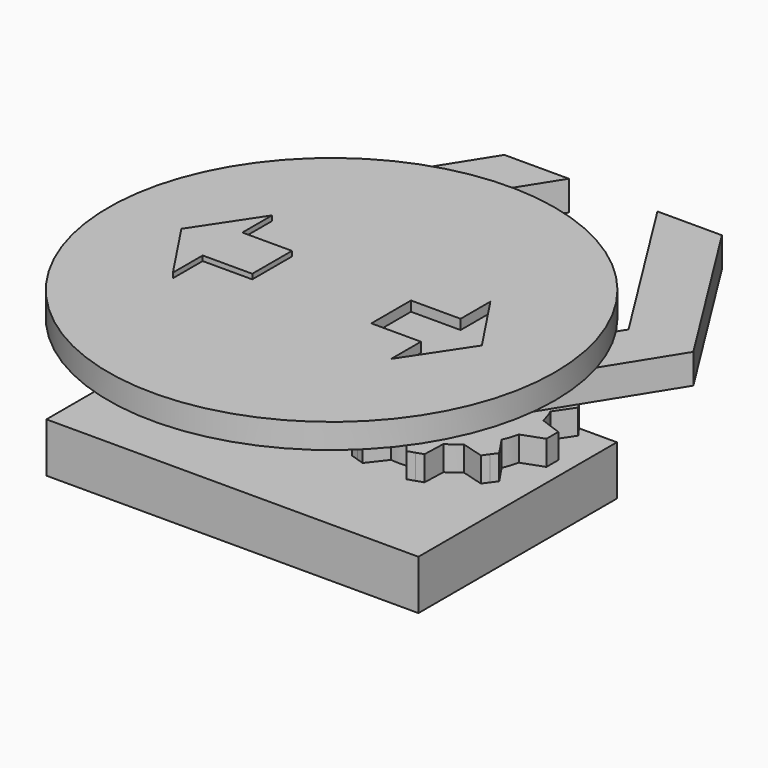
from build123d import *

# Parameters (mm, degrees)
F0_W      = 75
F0_H      = 50
F1_DEPTH  = 10
F2_R      = 10
F2_R_2    = 3.5
F3_DEPTH  = 2
F4_DEPTH  = 20
F5_DEPTH  = 20
F7_DEPTH  = 5
F9_DEPTH  = 5
F10_R     = 3.5
F11_DEPTH = 6
F13_R     = 45
F14_DEPTH = 5
F15_R     = 5
F15_R_2   = 3.5
F16_DEPTH = 7
F18_DEPTH = 2
F19_DEPTH = 3


with BuildPart() as f1:
    # F0 (on Top) → F1 (new body)
    with BuildSketch(Plane.XY):
        Rectangle(F0_W, F0_H)
    extrude(amount=F1_DEPTH)

    # F2 (on face) → F3 (join)
    with BuildSketch(Plane.XY.offset(10)):
        with Locations((-17.5, 10)):
            Circle(F2_R)
        with Locations((-17.5, 10)):
            Circle(F2_R_2, mode=Mode.SUBTRACT)
        with Locations((17.5, 10)):
            Circle(F2_R)
        with Locations((17.5, 10)):
            Circle(F2_R_2, mode=Mode.SUBTRACT)
    extrude(amount=F3_DEPTH)


with BuildPart() as f4:
    # F4 (new): a face of the model
    f4_faces = [f1.part.faces().sort_by_distance(p)[0] for p in [
        (-17.5, 10, 10),
    ]]
    extrude(f4_faces, amount=F4_DEPTH)

    # F6 (on face) → F7 (join)
    with BuildSketch(Plane.XY.offset(12)):
        with BuildLine():
            ThreePointArc((-2.587280565, 8.3842032761), (-2.521836035, 9.190923837), (-2.5, 10))
            ThreePointArc((-2.5, 10), (-2.521836035, 10.809076163), (-2.587280565, 11.6157967239))
            ThreePointArc((-2.587280565, 11.6157967239), (-3.2341522556, 14.6352549156), (-4.4856150597, 17.4582695463))
            ThreePointArc((-4.4856150597, 17.4582695463), (-5.3647450844, 18.8167787844), (-6.3850980298, 20.0726835646))
            ThreePointArc((-6.3850980298, 20.0726835646), (-8.6832212156, 22.1352549156), (-11.3550022589, 23.6835303472))
            ThreePointArc((-11.3550022589, 23.6835303472), (-12.8647450844, 24.2658477444), (-14.4284302655, 24.6821476415))
            ThreePointArc((-14.4284302655, 24.6821476415), (-17.5, 25), (-20.5715697345, 24.6821476415))
            ThreePointArc((-20.5715697345, 24.6821476415), (-22.1352549156, 24.2658477444), (-23.6449977411, 23.6835303472))
            ThreePointArc((-23.6449977411, 23.6835303472), (-26.3167787844, 22.1352549156), (-28.6149019702, 20.0726835646))
            ThreePointArc((-28.6149019702, 20.0726835646), (-29.6352549156, 18.8167787844), (-30.5143849403, 17.4582695463))
            ThreePointArc((-30.5143849403, 17.4582695463), (-31.7658477444, 14.6352549156), (-32.412719435, 11.6157967239))
            ThreePointArc((-32.412719435, 11.6157967239), (-32.5, 10), (-32.412719435, 8.3842032761))
            ThreePointArc((-32.412719435, 8.3842032761), (-31.7658477444, 5.3647450844), (-30.5143849403, 2.5417304537))
            ThreePointArc((-30.5143849403, 2.5417304537), (-29.6352549156, 1.1832212156), (-28.6149019702, -0.0726835646))
            ThreePointArc((-28.6149019702, -0.0726835646), (-26.3167787844, -2.1352549156), (-23.6449977411, -3.6835303472))
            ThreePointArc((-23.6449977411, -3.6835303472), (-22.1352549156, -4.2658477444), (-20.5715697345, -4.6821476415))
            ThreePointArc((-20.5715697345, -4.6821476415), (-17.5, -5), (-14.4284302655, -4.6821476415))
            ThreePointArc((-14.4284302655, -4.6821476415), (-12.8647450844, -4.2658477444), (-11.3550022589, -3.6835303472))
            ThreePointArc((-11.3550022589, -3.6835303472), (-8.6832212156, -2.1352549156), (-6.3850980298, -0.0726835646))
            ThreePointArc((-6.3850980298, -0.0726835646), (-5.3647450844, 1.1832212156), (-4.4856150597, 2.5417304537))
            ThreePointArc((-4.4856150597, 2.5417304537), (-3.2341522556, 5.3647450844), (-2.587280565, 8.3842032761))
        make_face()
        with BuildLine():
            ThreePointArc((-4.4856150597, 17.4582695463), (-3.2341522556, 14.6352549156), (-2.587280565, 11.6157967239))
            Line((-2.587280565, 11.6157967239), (1.0335993012, 14.4447381187))
            Line((1.0335993012, 14.4447381187), (0.5700738096, 15.8713228931))
            Line((0.5700738096, 15.8713228931), (0.106548318, 17.2979076676))
            Line((0.106548318, 17.2979076676), (-4.4856150597, 17.4582695463))
        make_face()
        with BuildLine():
            Line((1.0335993012, 5.5552618813), (-2.587280565, 8.3842032761))
            ThreePointArc((-2.587280565, 8.3842032761), (-3.2341522556, 5.3647450844), (-4.4856150597, 2.5417304537))
            Line((-4.4856150597, 2.5417304537), (0.106548318, 2.7020923324))
            Line((0.106548318, 2.7020923324), (0.5700738096, 4.1286771069))
            Line((0.5700738096, 4.1286771069), (1.0335993012, 5.5552618813))
        make_face()
        with BuildLine():
            ThreePointArc((-11.3550022589, 23.6835303472), (-8.6832212156, 22.1352549156), (-6.3850980298, 20.0726835646))
            Line((-6.3850980298, 20.0726835646), (-5.1185547149, 24.4896450147))
            Line((-5.1185547149, 24.4896450147), (-6.3320802064, 25.3713228931))
            Line((-6.3320802064, 25.3713228931), (-7.545605698, 26.2530007716))
            Line((-7.545605698, 26.2530007716), (-11.3550022589, 23.6835303472))
        make_face()
        with BuildLine():
            Line((-5.1185547149, -4.4896450147), (-6.3850980298, -0.0726835646))
            ThreePointArc((-6.3850980298, -0.0726835646), (-8.6832212156, -2.1352549156), (-11.3550022589, -3.6835303472))
            Line((-11.3550022589, -3.6835303472), (-7.545605698, -6.2530007716))
            Line((-7.545605698, -6.2530007716), (-6.3320802064, -5.3713228931))
            Line((-6.3320802064, -5.3713228931), (-5.1185547149, -4.4896450147))
        make_face()
        with BuildLine():
            ThreePointArc((-20.5715697345, 24.6821476415), (-17.5, 25), (-14.4284302655, 24.6821476415))
            Line((-14.4284302655, 24.6821476415), (-16, 29))
            Line((-16, 29), (-17.5, 29))
            Line((-17.5, 29), (-19, 29))
            Line((-19, 29), (-20.5715697345, 24.6821476415))
        make_face()
        with BuildLine():
            Line((-16, -9), (-14.4284302655, -4.6821476415))
            ThreePointArc((-14.4284302655, -4.6821476415), (-17.5, -5), (-20.5715697345, -4.6821476415))
            Line((-20.5715697345, -4.6821476415), (-19, -9))
            Line((-19, -9), (-17.5, -9))
            Line((-17.5, -9), (-16, -9))
        make_face()
        with BuildLine():
            ThreePointArc((-28.6149019702, 20.0726835646), (-26.3167787844, 22.1352549156), (-23.6449977411, 23.6835303472))
            Line((-23.6449977411, 23.6835303472), (-27.454394302, 26.2530007716))
            Line((-27.454394302, 26.2530007716), (-28.6679197936, 25.3713228931))
            Line((-28.6679197936, 25.3713228931), (-29.8814452851, 24.4896450147))
            Line((-29.8814452851, 24.4896450147), (-28.6149019702, 20.0726835646))
        make_face()
        with BuildLine():
            Line((-27.454394302, -6.2530007716), (-23.6449977411, -3.6835303472))
            ThreePointArc((-23.6449977411, -3.6835303472), (-26.3167787844, -2.1352549156), (-28.6149019702, -0.0726835646))
            Line((-28.6149019702, -0.0726835646), (-29.8814452851, -4.4896450147))
            Line((-29.8814452851, -4.4896450147), (-28.6679197936, -5.3713228931))
            Line((-28.6679197936, -5.3713228931), (-27.454394302, -6.2530007716))
        make_face()
        with BuildLine():
            ThreePointArc((-32.412719435, 11.6157967239), (-31.7658477444, 14.6352549156), (-30.5143849403, 17.4582695463))
            Line((-30.5143849403, 17.4582695463), (-35.106548318, 17.2979076676))
            Line((-35.106548318, 17.2979076676), (-35.5700738096, 15.8713228931))
            Line((-35.5700738096, 15.8713228931), (-36.0335993012, 14.4447381187))
            Line((-36.0335993012, 14.4447381187), (-32.412719435, 11.6157967239))
        make_face()
        with BuildLine():
            Line((-35.106548318, 2.7020923324), (-30.5143849403, 2.5417304537))
            ThreePointArc((-30.5143849403, 2.5417304537), (-31.7658477444, 5.3647450844), (-32.412719435, 8.3842032761))
            Line((-32.412719435, 8.3842032761), (-36.0335993012, 5.5552618813))
            Line((-36.0335993012, 5.5552618813), (-35.5700738096, 4.1286771069))
            Line((-35.5700738096, 4.1286771069), (-35.106548318, 2.7020923324))
        make_face()
    extrude(amount=F7_DEPTH)


with BuildPart() as f5:
    # F5 (new): a face of the model
    f5_faces = [f1.part.faces().sort_by_distance(p)[0] for p in [
        (17.5, 10, 10),
    ]]
    extrude(f5_faces, amount=F5_DEPTH)

    # F8 (on face) → F9 (join)
    with BuildSketch(Plane.XY.offset(12)):
        with BuildLine():
            ThreePointArc((32.1821476415, 6.9284302655), (32.4203253085, 8.4560140257), (32.5, 10))
            ThreePointArc((32.5, 10), (32.4203253085, 11.5439859743), (32.1821476415, 13.0715697345))
            ThreePointArc((32.1821476415, 13.0715697345), (31.7658477444, 14.6352549156), (31.1835303472, 16.1449977411))
            ThreePointArc((31.1835303472, 16.1449977411), (29.6352549156, 18.8167787844), (27.5726835646, 21.1149019702))
            ThreePointArc((27.5726835646, 21.1149019702), (26.3167787844, 22.1352549156), (24.9582695463, 23.0143849403))
            ThreePointArc((24.9582695463, 23.0143849403), (22.1352549156, 24.2658477444), (19.1157967239, 24.912719435))
            ThreePointArc((19.1157967239, 24.912719435), (17.5, 25), (15.8842032761, 24.912719435))
            ThreePointArc((15.8842032761, 24.912719435), (12.8647450844, 24.2658477444), (10.0417304537, 23.0143849403))
            ThreePointArc((10.0417304537, 23.0143849403), (8.6832212156, 22.1352549156), (7.4273164354, 21.1149019702))
            ThreePointArc((7.4273164354, 21.1149019702), (5.3647450844, 18.8167787844), (3.8164696528, 16.1449977411))
            ThreePointArc((3.8164696528, 16.1449977411), (3.2341522556, 14.6352549156), (2.8178523585, 13.0715697345))
            ThreePointArc((2.8178523585, 13.0715697345), (2.5, 10), (2.8178523585, 6.9284302655))
            ThreePointArc((2.8178523585, 6.9284302655), (3.2341522556, 5.3647450844), (3.8164696528, 3.8550022589))
            ThreePointArc((3.8164696528, 3.8550022589), (5.3647450844, 1.1832212156), (7.4273164354, -1.1149019702))
            ThreePointArc((7.4273164354, -1.1149019702), (8.6832212156, -2.1352549156), (10.0417304537, -3.0143849403))
            ThreePointArc((10.0417304537, -3.0143849403), (12.8647450844, -4.2658477444), (15.8842032761, -4.912719435))
            ThreePointArc((15.8842032761, -4.912719435), (17.5, -5), (19.1157967239, -4.912719435))
            ThreePointArc((19.1157967239, -4.912719435), (22.1352549156, -4.2658477444), (24.9582695463, -3.0143849403))
            ThreePointArc((24.9582695463, -3.0143849403), (26.3167787844, -2.1352549156), (27.5726835646, -1.1149019702))
            ThreePointArc((27.5726835646, -1.1149019702), (29.6352549156, 1.1832212156), (31.1835303472, 3.8550022589))
            ThreePointArc((31.1835303472, 3.8550022589), (31.7658477444, 5.3647450844), (32.1821476415, 6.9284302655))
        make_face()
        with BuildLine():
            ThreePointArc((32.1821476415, 13.0715697345), (32.4203253085, 11.5439859743), (32.5, 10))
            ThreePointArc((32.5, 10), (32.4203253085, 8.4560140257), (32.1821476415, 6.9284302655))
            Line((32.1821476415, 6.9284302655), (36.5, 8.5))
            Line((36.5, 8.5), (36.5, 10))
            Line((36.5, 10), (36.5, 11.5))
            Line((36.5, 11.5), (32.1821476415, 13.0715697345))
        make_face()
        with BuildLine():
            ThreePointArc((27.5726835646, 21.1149019702), (29.6352549156, 18.8167787844), (31.1835303472, 16.1449977411))
            Line((31.1835303472, 16.1449977411), (33.7530007716, 19.954394302))
            Line((33.7530007716, 19.954394302), (32.8713228931, 21.1679197936))
            Line((32.8713228931, 21.1679197936), (31.9896450147, 22.3814452851))
            Line((31.9896450147, 22.3814452851), (27.5726835646, 21.1149019702))
        make_face()
        with BuildLine():
            Line((33.7530007716, 0.045605698), (31.1835303472, 3.8550022589))
            ThreePointArc((31.1835303472, 3.8550022589), (29.6352549156, 1.1832212156), (27.5726835646, -1.1149019702))
            Line((27.5726835646, -1.1149019702), (31.9896450147, -2.3814452851))
            Line((31.9896450147, -2.3814452851), (32.8713228931, -1.1679197936))
            Line((32.8713228931, -1.1679197936), (33.7530007716, 0.045605698))
        make_face()
        with BuildLine():
            ThreePointArc((19.1157967239, 24.912719435), (22.1352549156, 24.2658477444), (24.9582695463, 23.0143849403))
            Line((24.9582695463, 23.0143849403), (24.7979076676, 27.606548318))
            Line((24.7979076676, 27.606548318), (23.3713228931, 28.0700738096))
            Line((23.3713228931, 28.0700738096), (21.9447381187, 28.5335993012))
            Line((21.9447381187, 28.5335993012), (19.1157967239, 24.912719435))
        make_face()
        with BuildLine():
            Line((24.7979076676, -7.606548318), (24.9582695463, -3.0143849403))
            ThreePointArc((24.9582695463, -3.0143849403), (22.1352549156, -4.2658477444), (19.1157967239, -4.912719435))
            Line((19.1157967239, -4.912719435), (21.9447381187, -8.5335993012))
            Line((21.9447381187, -8.5335993012), (23.3713228931, -8.0700738096))
            Line((23.3713228931, -8.0700738096), (24.7979076676, -7.606548318))
        make_face()
        with BuildLine():
            ThreePointArc((10.0417304537, 23.0143849403), (12.8647450844, 24.2658477444), (15.8842032761, 24.912719435))
            Line((15.8842032761, 24.912719435), (13.0552618813, 28.5335993012))
            Line((13.0552618813, 28.5335993012), (11.6286771069, 28.0700738096))
            Line((11.6286771069, 28.0700738096), (10.2020923324, 27.606548318))
            Line((10.2020923324, 27.606548318), (10.0417304537, 23.0143849403))
        make_face()
        with BuildLine():
            Line((13.0552618813, -8.5335993012), (15.8842032761, -4.912719435))
            ThreePointArc((15.8842032761, -4.912719435), (12.8647450844, -4.2658477444), (10.0417304537, -3.0143849403))
            Line((10.0417304537, -3.0143849403), (10.2020923324, -7.606548318))
            Line((10.2020923324, -7.606548318), (11.6286771069, -8.0700738096))
            Line((11.6286771069, -8.0700738096), (13.0552618813, -8.5335993012))
        make_face()
        with BuildLine():
            ThreePointArc((3.8164696528, 16.1449977411), (5.3647450844, 18.8167787844), (7.4273164354, 21.1149019702))
            Line((7.4273164354, 21.1149019702), (3.0103549853, 22.3814452851))
            Line((3.0103549853, 22.3814452851), (2.1286771069, 21.1679197936))
            Line((2.1286771069, 21.1679197936), (1.2469992284, 19.954394302))
            Line((1.2469992284, 19.954394302), (3.8164696528, 16.1449977411))
        make_face()
        with BuildLine():
            Line((3.0103549853, -2.3814452851), (7.4273164354, -1.1149019702))
            ThreePointArc((7.4273164354, -1.1149019702), (5.3647450844, 1.1832212156), (3.8164696528, 3.8550022589))
            Line((3.8164696528, 3.8550022589), (1.2469992284, 0.045605698))
            Line((1.2469992284, 0.045605698), (2.1286771069, -1.1679197936))
            Line((2.1286771069, -1.1679197936), (3.0103549853, -2.3814452851))
        make_face()
        with BuildLine():
            ThreePointArc((2.8178523585, 6.9284302655), (2.5, 10), (2.8178523585, 13.0715697345))
            Line((2.8178523585, 13.0715697345), (-1.5, 11.5))
            Line((-1.5, 11.5), (-1.5, 10))
            Line((-1.5, 10), (-1.5, 8.5))
            Line((-1.5, 8.5), (2.8178523585, 6.9284302655))
        make_face()
    extrude(amount=F9_DEPTH)


with BuildPart() as f11:
    # F10 (on face) → F11 (new body)
    with BuildSketch(Plane.XY.offset(17)):
        with BuildLine():
            ThreePointArc((-27.3644237339, 11.6410802534), (-18.3233354909, 0.0339517024), (-7.5, 10))
            ThreePointArc((-7.5, 10), (-11.3458917676, 17.8820652029), (-19.9253903727, 19.7014164708))
            ThreePointArc((-19.9253903727, 19.7014164708), (-24.8486146775, 16.7821723896), (-27.3644237339, 11.6410802534))
        make_face()
        with Locations((-17.5, 10)):
            Circle(F10_R, mode=Mode.SUBTRACT)
        with BuildLine():
            ThreePointArc((-27.3644237339, 11.6410802534), (-24.8486146775, 16.7821723896), (-19.9253903727, 19.7014164708))
            Line((-19.9253903727, 19.7014164708), (-30.5143849403, 36.6682427517))
            Line((-30.5143849403, 36.6682427517), (-8.9303671844, 70.937473521))
            Line((-8.9303671844, 70.937473521), (-21.9303671844, 70.937473521))
            Line((-21.9303671844, 70.937473521), (-43.2479155853, 37.0913196748))
            Line((-43.2479155853, 37.0913196748), (-27.3644237339, 11.6410802534))
        make_face()
    extrude(amount=F11_DEPTH)


with BuildPart() as f12_1:
    # F12: instance of F11
    add(f11.part.mirror(Plane.YZ))


with BuildPart() as f14:
    # F13 (on face) → F14 (new body)
    with BuildSketch(Plane.XY.offset(30)):
        Circle(F13_R)
    extrude(amount=F14_DEPTH)

    # F15 (on face) → F16 (join, through all)
    with BuildSketch(Plane(origin=(0, 0, 30), x_dir=(1, 0, 0), z_dir=(0, 0, -1))):
        with Locations((-17.5, -10)):
            Circle(F15_R)
        with Locations((-17.5, -10)):
            Circle(F15_R_2, mode=Mode.SUBTRACT)
        with Locations((17.5, -10)):
            Circle(F15_R)
        with Locations((17.5, -10)):
            Circle(F15_R_2, mode=Mode.SUBTRACT)
    extrude(amount=F16_DEPTH)

    # F17 (on face) → F18 (cut)
    with BuildSketch(Plane.XY.offset(35)):
        Polygon((-12, -5), (-12, 0), (-12, 5), (-22, 5), (-22, 12.5), (-30.2915619759, 0), (-22, -12.5), (-22, -5), align=None)
        Polygon((12, 5), (12, 0), (12, -5), (22, -5), (22, -12.5), (30.2915619759, 0), (22, 12.5), (22, 5), align=None)
    extrude(amount=-F18_DEPTH, mode=Mode.SUBTRACT)


with BuildPart() as f19:
    # F19 (new): a face of the model
    f19_faces = [f14.part.faces().sort_by_distance(p)[0] for p in [
        (-20.9513999113, 0, 33),
    ]]
    extrude(f19_faces, amount=F19_DEPTH)


solid = Compound([f1.part, f4.part, f5.part, f11.part, f12_1.part, f14.part, f19.part])
